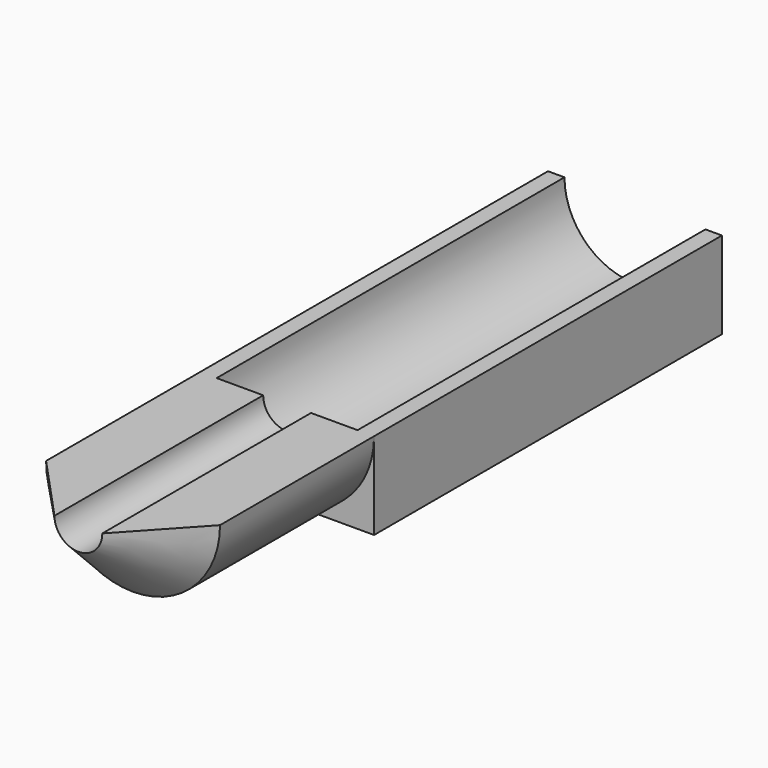
from build123d import *

# Parameters (mm, degrees)
F0_W     = 0.7586409766
F0_H     = 4.9999998882
F0_H_2   = 9
F0_H_3   = 6.0000001118
F1_ANGLE = 180
F3_DEPTH = 20


with BuildPart() as f1:
    # F0 (on Top) → F1 (revolve)
    with BuildSketch(Plane.XY):
        Polygon((-4, -8.8572846726), (-1.1, -12), (-1.1, 0), (-1.55, 0), (-3.2413590234, 0), (-4, 0), align=None)
        with Locations((-3.6206795117, 2.4999999441)):
            Rectangle(F0_W, F0_H)
        with Locations((-3.6206795117, 9.4999998882)):
            Rectangle(F0_W, F0_H_2)
        with Locations((-3.6206795117, 16.9999999441)):
            Rectangle(F0_W, F0_H_3)
    revolve(axis=Axis((0, 4.4247480631, 0), (0, -1, 0)), revolution_arc=F1_ANGLE)

    # F2 (on face) → F3 (join)
    with BuildSketch(Plane(origin=(0, 20, 0), x_dir=(-1, 0, 0), z_dir=(0, 1, 0))):
        with BuildLine():
            ThreePointArc((0, -4), (-2.8284271247, -2.8284271247), (-4, 0))
            Line((-4, 0), (-4, -4))
            Line((-4, -4), (0, -4))
        make_face()
        with BuildLine():
            ThreePointArc((4, 0), (2.8284271247, -2.8284271247), (0, -4))
            Line((0, -4), (4, -4))
            Line((4, -4), (4, 0))
        make_face()
    extrude(amount=-F3_DEPTH)


solid = f1.part
